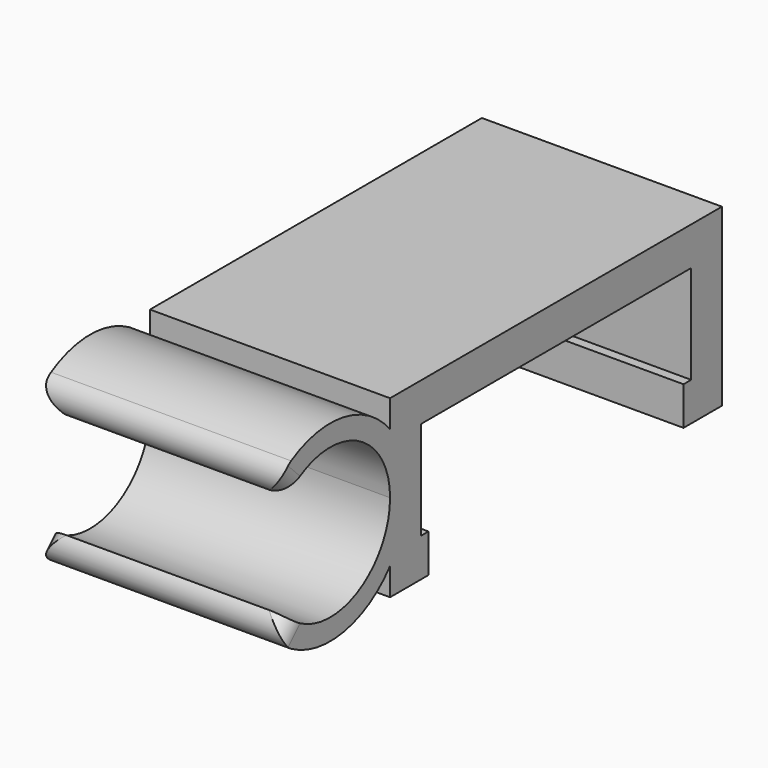
from build123d import *

# Parameters (mm, degrees)
F1_DEPTH    = 25
F2_DEPTH    = 25
F3_T1_DEPTH = 12.2
F3_T3_DEPTH = 12.2
F3_T5_DEPTH = 12.2
F3_T7_DEPTH = 12.2
F4_T1_DEPTH = 33.6004292483


# Not quite as in the source:
# - a fillet or chamfer that OpenCascade refuses, or shapes differently, is made with other operations: its cross-section is extruded or revolved along the edge and cut away or added


with BuildPart() as f1:
    # F0 (on Right) → F1 (new body)
    with BuildSketch(Plane.YZ):
        with BuildLine():
            Line((17.6, 0.1), (17.6, -10.15))
            Line((17.6, -10.15), (16.6, -10.15))
            Line((16.6, -10.15), (16.6, -14.15))
            Line((16.6, -14.15), (21.6, -14.15))
            Line((21.6, -14.15), (21.6, 4.1))
            Line((21.6, 4.1), (0, 4.1))
            Line((0, 4.1), (-21.6, 4.1))
            Line((-21.6, 4.1), (-21.6, 1.2327951389))
            ThreePointArc((-21.6, 1.2327951389), (-19.9660188679, -1.7083752096), (-19.4, -5.025))
            ThreePointArc((-19.4, -5.025), (-19.9660188679, -8.3416247904), (-21.6, -11.2827951389))
            Line((-21.6, -11.2827951389), (-21.6, -14.15))
            Line((-21.6, -14.15), (-16.6, -14.15))
            Line((-16.6, -14.15), (-16.6, -10.15))
            Line((-16.6, -10.15), (-17.6, -10.15))
            Line((-17.6, -10.15), (-17.6, 0.1))
            Line((-17.6, 0.1), (0, 0.1))
            Line((0, 0.1), (17.6, 0.1))
        make_face()
    extrude(amount=F1_DEPTH)

    # F0 (on Right) → F2 (join)
    with BuildSketch(Plane.YZ):
        with BuildLine():
            Line((-21.6, -5.025), (-21.6, 1.2327951389))
            ThreePointArc((-21.6, 1.2327951389), (-28.8539334803, 4.9600794366), (-36.4710678119, 2.0460678119))
            Line((-36.4710678119, 2.0460678119), (-34.9154328933, 0.4904328933))
            ThreePointArc((-34.9154328933, 0.4904328933), (-26.4150692276, 2.1812603536), (-21.6, -5.025))
        make_face()
        with BuildLine():
            Line((-21.6, -11.2827951389), (-21.6, -5.025))
            ThreePointArc((-21.6, -5.025), (-26.4150692276, -12.2312603536), (-34.9154328933, -10.5404328933))
            Line((-34.9154328933, -10.5404328933), (-36.4710678119, -12.0960678119))
            ThreePointArc((-36.4710678119, -12.0960678119), (-28.8539334803, -15.0100794366), (-21.6, -11.2827951389))
        make_face()
        with BuildLine():
            ThreePointArc((-19.4, -5.025), (-19.9660188679, -1.7083752096), (-21.6, 1.2327951389))
            Line((-21.6, 1.2327951389), (-21.6, -5.025))
            Line((-21.6, -5.025), (-21.6, -11.2827951389))
            ThreePointArc((-21.6, -11.2827951389), (-19.9660188679, -8.3416247904), (-19.4, -5.025))
        make_face()
    extrude(amount=F2_DEPTH)

    # F3: fillet of radius 2 on 4 edges, made by hand

    # F3_s2 → F3_t1 (cut)
    with BuildSketch(Plane(origin=(0, -19.1923989873, -19.1923989873), x_dir=(1, 0, 0), z_dir=(0, -0.7071067812, -0.7071067812))):
        with BuildLine():
            ThreePointArc((23, 17.2357277914), (24.4142135624, 16.6499413538), (25, 15.2357277914))
            Line((25, 15.2357277914), (25, 17.2357277914))
            Line((25, 17.2357277914), (23, 17.2357277914))
        make_face()
    extrude(amount=F3_T1_DEPTH, mode=Mode.SUBTRACT)

    # F3_s4 → F3_t3 (cut)
    with BuildSketch(Plane(origin=(0, -19.1923989873, -19.1923989873), x_dir=(1, 0, 0), z_dir=(0, -0.7071067812, -0.7071067812))):
        with BuildLine():
            ThreePointArc((0, 15.2357277914), (0.5857864376, 16.6499413538), (2, 17.2357277914))
            Line((2, 17.2357277914), (0, 17.2357277914))
            Line((0, 17.2357277914), (0, 15.2357277914))
        make_face()
    extrude(amount=F3_T3_DEPTH, mode=Mode.SUBTRACT)

    # F3_s6 → F3_t5 (cut)
    with BuildSketch(Plane(origin=(0, -22.7941017178, 22.7941017178), x_dir=(1, 0, 0), z_dir=(0, 0.7071067812, -0.7071067812))):
        with BuildLine():
            ThreePointArc((25, 22.3421509423), (24.4142135624, 23.7563645047), (23, 24.3421509423))
            Line((23, 24.3421509423), (25, 24.3421509423))
            Line((25, 24.3421509423), (25, 22.3421509423))
        make_face()
    extrude(amount=F3_T5_DEPTH, mode=Mode.SUBTRACT)

    # F3_s8 → F3_t7 (cut)
    with BuildSketch(Plane(origin=(0, -22.7941017178, 22.7941017178), x_dir=(1, 0, 0), z_dir=(0, 0.7071067812, -0.7071067812))):
        with BuildLine():
            ThreePointArc((0, 22.3421509423), (0.5857864376, 23.7563645047), (2, 24.3421509423))
            Line((2, 24.3421509423), (0, 24.3421509423))
            Line((0, 24.3421509423), (0, 22.3421509423))
        make_face()
    extrude(amount=F3_T7_DEPTH, mode=Mode.SUBTRACT)

    # F4: fillet of radius 2 on 2 edges, made by hand

    # F4_s2 → F4_t1 (cut)
    with BuildSketch(Plane.YZ.offset(-4.3002146241)):
        with BuildLine():
            ThreePointArc((-34.8772255751, 0.4522255751), (-35.4470714052, 2.1184477224), (-34.4787650158, 3.5892989218))
            ThreePointArc((-34.4787650158, 3.5892989218), (-35.523724357, 2.8806941504), (-36.4710678119, 2.0460678119))
            Line((-36.4710678119, 2.0460678119), (-34.8772255751, 0.4522255751))
        make_face()
        with BuildLine():
            ThreePointArc((-34.8772255751, -10.5022255751), (-35.4470714052, -12.1684477224), (-34.4787650158, -13.6392989218))
            ThreePointArc((-34.4787650158, -13.6392989218), (-35.523724357, -12.9306941504), (-36.4710678119, -12.0960678119))
            Line((-36.4710678119, -12.0960678119), (-34.8772255751, -10.5022255751))
        make_face()
    extrude(amount=F4_T1_DEPTH, mode=Mode.SUBTRACT)


solid = f1.part
